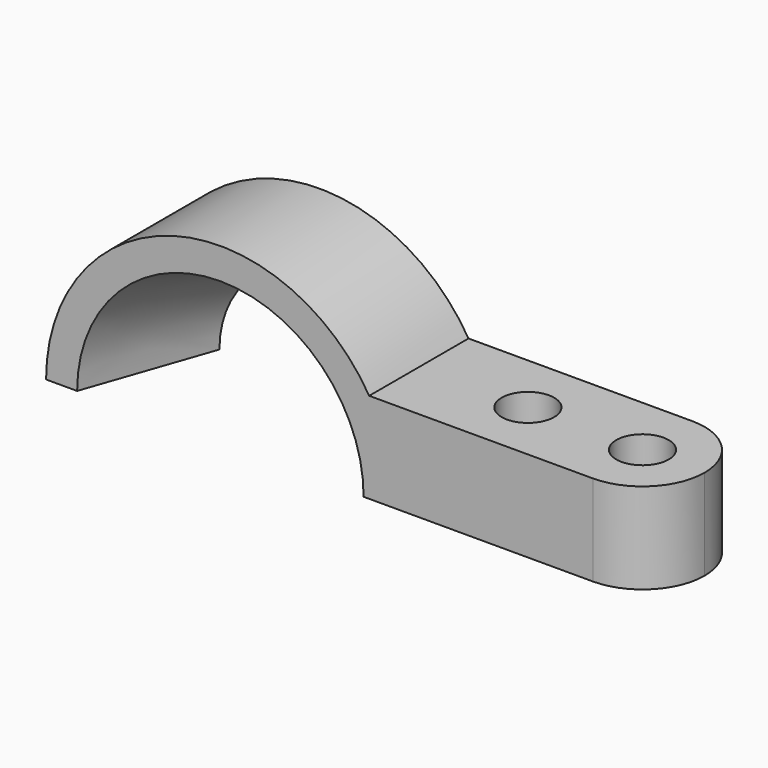
from build123d import *

# Parameters (mm, degrees)
F1_DEPTH = 52
F4_R     = 11
F5_DEPTH = 77
F6_R     = 25.99999


# Not quite as in the source:
# - a fillet or chamfer is up to 0.001 mm smaller than in the source, because OpenCascade refuses the exact size


with BuildPart() as f1:
    # F0 (on Front) → F1 (new body)
    with BuildSketch(Plane.XZ):
        with BuildLine():
            Line((182, 38), (62.329768169, 38))
            ThreePointArc((62.329768169, 38), (-19.7348286497, 70.2818364741), (-73, 0))
            Line((-73, 0), (182, 0))
            Line((182, 0), (182, 38))
        make_face()
    extrude(amount=F1_DEPTH)

    # F2 (on face) → F3 (revolve, cut)
    with BuildSketch(Plane(origin=(0, 0, 0), x_dir=(1, 0, 0), z_dir=(0, 0, -1))):
        Polygon((0, 52), (-60, 52), (-42, 0), (0, 0), align=None)
    revolve(axis=Axis((0, -26, 0), (0, -1, 0)), mode=Mode.SUBTRACT)

    # F4 (on face) → F5 (cut)
    with BuildSketch(Plane(origin=(0, 0, 0), x_dir=(1, 0, 0), z_dir=(0, 0, -1))):
        with Locations((108, 26)):
            Circle(F4_R)
        with Locations((156, 26)):
            Circle(F4_R)
    extrude(amount=-F5_DEPTH, mode=Mode.SUBTRACT)

    # F6 (radius 26 in the source; OpenCascade refuses exactly that, so slightly less here)
    f6_edges = [f1.edges().sort_by_distance(p)[0] for p in [
        (182, -52, 19),
        (182, 0, 19),
    ]]
    fillet(f6_edges, radius=F6_R)


solid = f1.part
